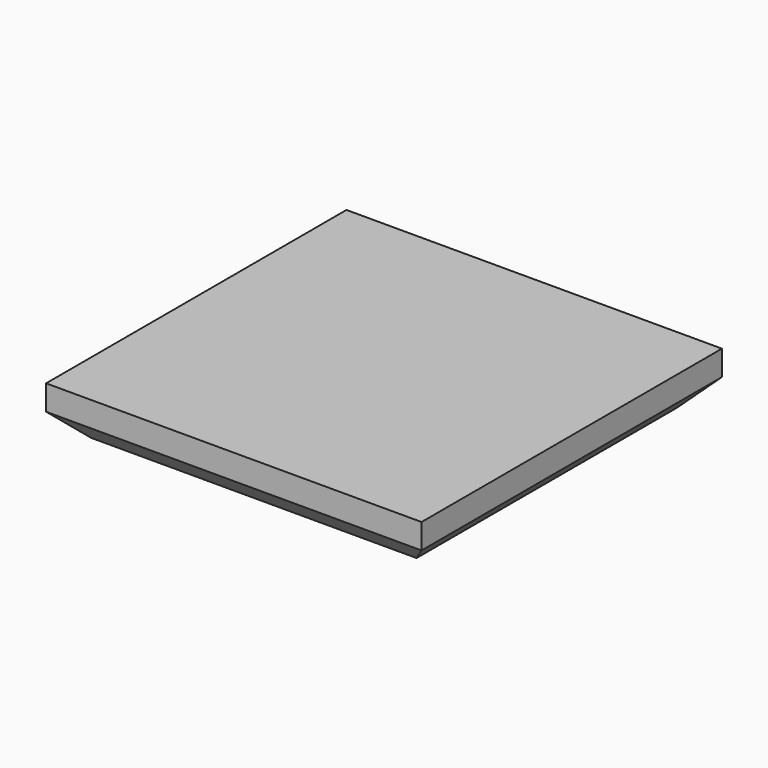
from build123d import *

# Parameters (mm, degrees)
F0_W     = 76.2
F0_H     = 76.2
F1_DEPTH = 10.16
F2_SIZE  = 5.08


# Not quite as in the source:
# - the program builds the solid bodies; features that only make, move or delete a surface that nothing else refers to are left out


with BuildPart() as f1:
    # F0 (on Top) → F1 (new body)
    with BuildSketch(Plane.XY):
        Rectangle(F0_W, F0_H)
    extrude(amount=F1_DEPTH)

    # F2
    f2_edges = [f1.edges().sort_by_distance(p)[0] for p in [
        (0, 38.1, 0),
        (38.1, 0, 0),
        (0, -38.1, 0),
        (-38.1, 0, 0),
    ]]
    chamfer(f2_edges, length=F2_SIZE)


solid = f1.part
